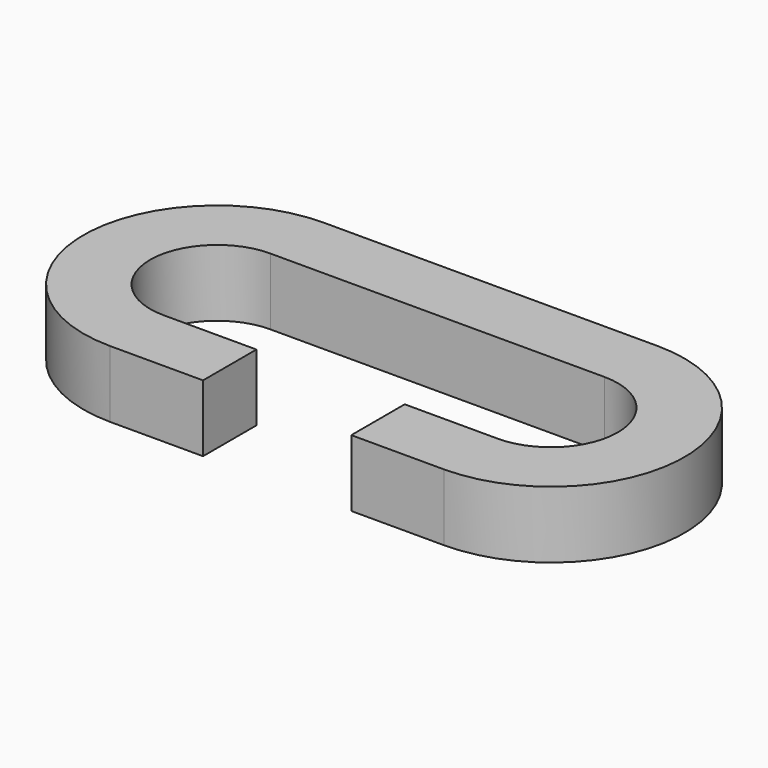
from build123d import *

# Parameters (mm, degrees)
F1_DEPTH = 12.7


# Not quite as in the source:
# - a feature of the source that left no trace in its solid (it failed there, or was rolled back) is left out


with BuildPart() as f1:
    # F0 (on Top) → F1 (new body)
    with BuildSketch(Plane.XY):
        with BuildLine():
            ThreePointArc((31.75, 12.7), (44.45, 0), (31.75, -12.7))
            Line((31.75, -12.7), (14.0969706699, -12.7))
            Line((14.0969706699, -12.7), (14.0969706699, -25.4))
            Line((14.0969706699, -25.4), (31.75, -25.4))
            ThreePointArc((31.75, -25.4), (57.15, 0), (31.75, 25.4))
            Line((31.75, 25.4), (0, 25.4))
            Line((0, 25.4), (-31.75, 25.4))
            ThreePointArc((-31.75, 25.4), (-57.15, 0), (-31.75, -25.4))
            Line((-31.75, -25.4), (-14.0969706699, -25.4))
            Line((-14.0969706699, -25.4), (-14.0969706699, -12.7))
            Line((-14.0969706699, -12.7), (-31.75, -12.7))
            ThreePointArc((-31.75, -12.7), (-44.45, 0), (-31.75, 12.7))
            Line((-31.75, 12.7), (0, 12.7))
            Line((0, 12.7), (31.75, 12.7))
        make_face()
    extrude(amount=F1_DEPTH)


solid = f1.part
